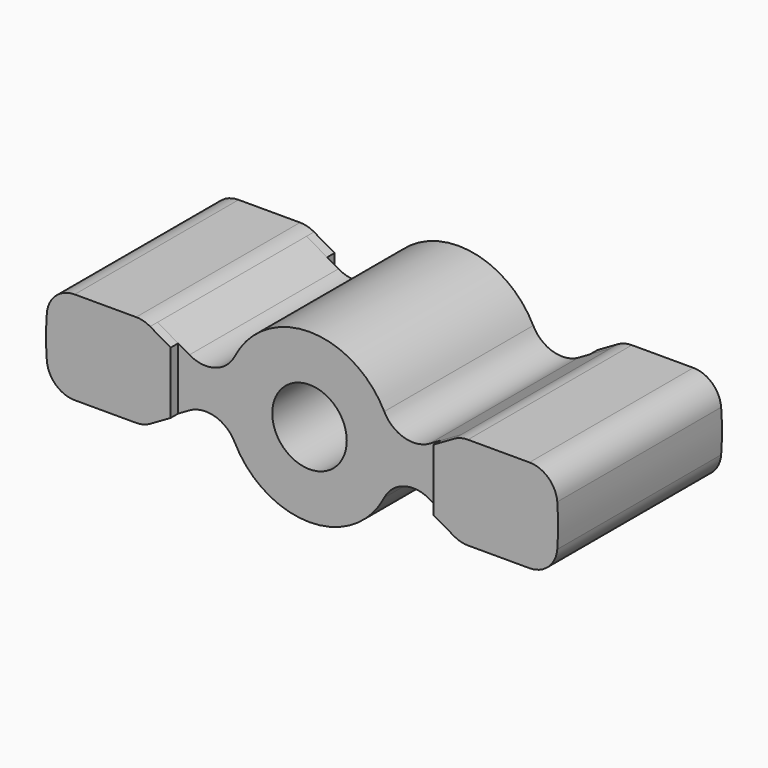
from build123d import *

# Parameters (mm, degrees)
F0_R     = 4
F1_DEPTH = 10
F3_DEPTH = 1


# Not quite as in the source:
# - a pattern or mirror of a feature is missing from the dataset's text; its kind, count and spacing are read off the source's solid


with BuildPart() as f1:
    # F0 (on Front) → F1 (new body, symmetric)
    with BuildSketch(Plane.XZ):
        with BuildLine():
            ThreePointArc((-12.8973712231, -2.6245379145), (-10.1504183848, -2.3006178802), (-8.0261072806, -4.072051316))
            ThreePointArc((-8.0261072806, -4.072051316), (0, -9), (8.0261072806, -4.072051316))
            ThreePointArc((8.0261072806, -4.072051316), (10.1504183848, -2.3006178802), (12.8973712231, -2.6245379145))
            Line((12.8973712231, -2.6245379145), (16.315639824, -4.5980762114))
            ThreePointArc((16.315639824, -4.5980762114), (17.0391826887, -4.8977774789), (17.815639824, -5))
            Line((17.815639824, -5), (24.4182308941, -5))
            ThreePointArc((24.4182308941, -5), (26.4511236757, -4.2062064588), (27.4082183506, -2.2448979592))
            ThreePointArc((27.4082183506, -2.2448979592), (27.5, 0), (27.4082183506, 2.2448979592))
            ThreePointArc((27.4082183506, 2.2448979592), (26.4511236757, 4.2062064588), (24.4182308941, 5))
            Line((24.4182308941, 5), (17.815639824, 5))
            ThreePointArc((17.815639824, 5), (17.0391826887, 4.8977774789), (16.315639824, 4.5980762114))
            Line((16.315639824, 4.5980762114), (12.8973712231, 2.6245379145))
            ThreePointArc((12.8973712231, 2.6245379145), (10.1504183848, 2.3006178802), (8.0261072806, 4.072051316))
            ThreePointArc((8.0261072806, 4.072051316), (0, 9), (-8.0261072806, 4.072051316))
            ThreePointArc((-8.0261072806, 4.072051316), (-10.1504183848, 2.3006178802), (-12.8973712231, 2.6245379145))
            Line((-12.8973712231, 2.6245379145), (-16.315639824, 4.5980762114))
            ThreePointArc((-16.315639824, 4.5980762114), (-17.0391826887, 4.8977774789), (-17.815639824, 5))
            Line((-17.815639824, 5), (-24.4182308941, 5))
            ThreePointArc((-24.4182308941, 5), (-26.4511236757, 4.2062064588), (-27.4082183506, 2.2448979592))
            ThreePointArc((-27.4082183506, 2.2448979592), (-27.5, 0), (-27.4082183506, -2.2448979592))
            ThreePointArc((-27.4082183506, -2.2448979592), (-26.4511236757, -4.2062064588), (-24.4182308941, -5))
            Line((-24.4182308941, -5), (-17.815639824, -5))
            ThreePointArc((-17.815639824, -5), (-17.0391826887, -4.8977774789), (-16.315639824, -4.5980762114))
            Line((-16.315639824, -4.5980762114), (-12.8973712231, -2.6245379145))
        make_face()
        Circle(F0_R, mode=Mode.SUBTRACT)
    extrude(amount=F1_DEPTH, both=True)

    # F2 (on face) → F3 (join)
    with BuildSketch(Plane.XZ.offset(10)):
        with BuildLine():
            Line((-24.4182308941, -5), (-17.815639824, -5))
            ThreePointArc((-17.815639824, -5), (-17.0391826887, -4.8977774789), (-16.315639824, -4.5980762114))
            Line((-16.315639824, -4.5980762114), (-14.1075365245, -3.323227177))
            Line((-14.1075365245, -3.323227177), (-14.1075365245, 3.323227177))
            Line((-14.1075365245, 3.323227177), (-16.315639824, 4.5980762114))
            ThreePointArc((-16.315639824, 4.5980762114), (-17.0391826887, 4.8977774789), (-17.815639824, 5))
            Line((-17.815639824, 5), (-24.4182308941, 5))
            ThreePointArc((-24.4182308941, 5), (-26.4511236757, 4.2062064588), (-27.4082183506, 2.2448979592))
            ThreePointArc((-27.4082183506, 2.2448979592), (-27.5, 0), (-27.4082183506, -2.2448979592))
            ThreePointArc((-27.4082183506, -2.2448979592), (-26.4511236757, -4.2062064588), (-24.4182308941, -5))
        make_face()
        with BuildLine():
            Line((14.1075365245, -3.323227177), (16.315639824, -4.5980762114))
            ThreePointArc((16.315639824, -4.5980762114), (17.0391826887, -4.8977774789), (17.815639824, -5))
            Line((17.815639824, -5), (24.4182308941, -5))
            ThreePointArc((24.4182308941, -5), (26.4511236757, -4.2062064588), (27.4082183506, -2.2448979592))
            ThreePointArc((27.4082183506, -2.2448979592), (27.5, 0), (27.4082183506, 2.2448979592))
            ThreePointArc((27.4082183506, 2.2448979592), (26.4511236757, 4.2062064588), (24.4182308941, 5))
            Line((24.4182308941, 5), (17.815639824, 5))
            ThreePointArc((17.815639824, 5), (17.0391826887, 4.8977774789), (16.315639824, 4.5980762114))
            Line((16.315639824, 4.5980762114), (14.1075365245, 3.323227177))
            Line((14.1075365245, 3.323227177), (14.1075365245, -3.323227177))
        make_face()
    f3 = extrude(amount=F3_DEPTH)

    # F3_copies: F3 across plane
    add(f3.mirror(Plane.ZX))


solid = f1.part
